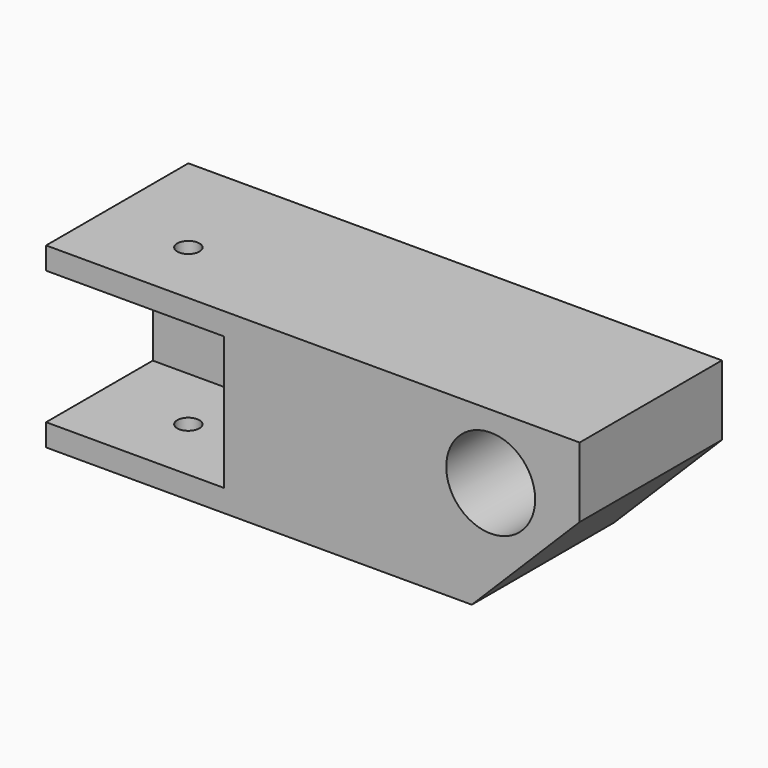
from build123d import *

# Parameters (mm, degrees)
F1_DEPTH = 50.8
F2_W     = 12.7
F2_H     = 38.1
F3_DEPTH = 50.8
F5_D     = 25.4
F7_D     = 6.35


# Not quite as in the source:
# - a feature names something its author has since deleted; it is built from what else it names


with BuildPart() as f1:
    # F0 (on Front) → F1 (new body)
    with BuildSketch(Plane.XZ):
        Polygon((-140.8084735786, 36.6746302678), (-140.8084735786, 30.3246302678), (-90.0084735786, 30.3246302678), (-90.0084735786, -7.7753697322), (-140.8084735786, -7.7753697322), (-140.8084735786, -14.1253697322), (-19.2084735786, -14.1253697322), (11.5915264214, 16.6746302678), (11.5915264214, 36.6746302678), align=None)
    extrude(amount=F1_DEPTH)

    # F2 (on face) → F3 (join)
    with BuildSketch(Plane(origin=(-90.0084735786, 0, 0), x_dir=(0, -1, 0), z_dir=(-1, 0, 0))):
        with Locations((6.35, 11.2746302678)):
            Rectangle(F2_W, F2_H)
    extrude(amount=F3_DEPTH)

    # F5 (through all)
    with Locations(Plane(origin=(0, 0, 0), x_dir=(-1, 0, 0), z_dir=(0, 1, 0))):
        with Locations((13.8084735786, 18.215398631)):
            Hole(F5_D / 2)

    # F7 (through all)
    with Locations(Plane.XY.offset(36.6746302678)):
        with Locations((-115.4084735786, -31.75)):
            Hole(F7_D / 2)


solid = f1.part
